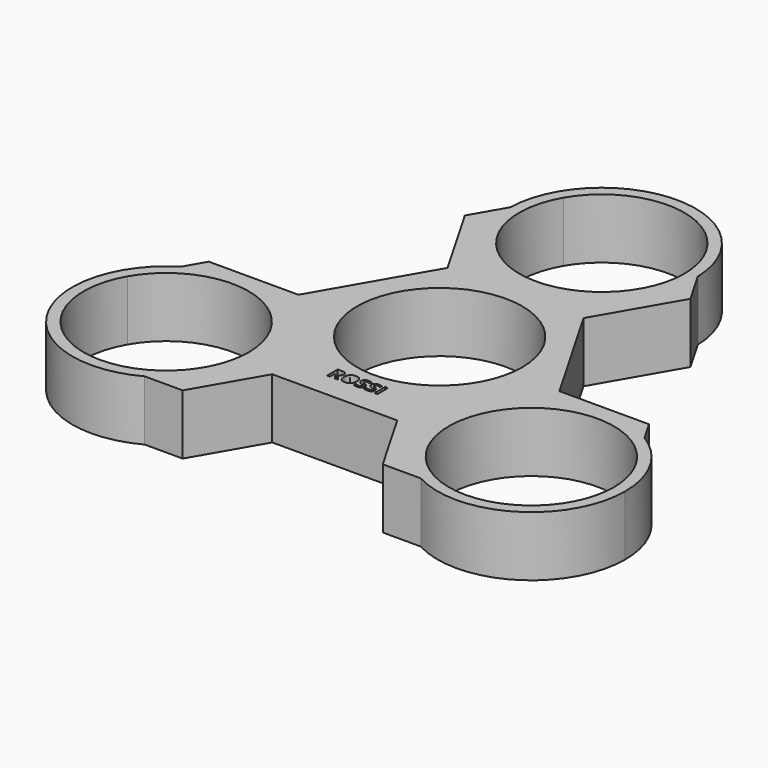
from build123d import *

# Parameters (mm, degrees)
F0_W     = 0.3740603024
F0_H     = 1.7637580204
F0_R     = 11
F1_DEPTH = 8


with BuildPart() as f1:
    # F0 (on Top) → F1 (new body)
    with BuildSketch(Plane.XY):
        with BuildLine():
            ThreePointArc((9.5262794416, 32.5), (10.6251840892, 29.8470094961), (11, 27))
            ThreePointArc((11, 27), (-2.8470094961, 16.3748159108), (-9.5262794416, 32.5))
            Line((-9.5262794416, 32.5), (-12.4948649634, 27.3582590497))
            ThreePointArc((-12.4948649634, 27.3582590497), (-0.1791479244, 14.5012838251), (12.5, 27))
            ThreePointArc((12.5, 27), (12.4987161749, 27.1791479244), (12.4948649634, 27.3582590497))
            Line((12.4948649634, 27.3582590497), (9.5262794416, 32.5))
        make_face()
        with BuildLine():
            ThreePointArc((-9.5262794416, 32.5), (0, 38), (9.5262794416, 32.5))
            Line((9.5262794416, 32.5), (12.4948649634, 27.3582590497))
            ThreePointArc((12.4948649634, 27.3582590497), (0, 39.5), (-12.4948649634, 27.3582590497))
            Line((-12.4948649634, 27.3582590497), (-9.5262794416, 32.5))
        make_face()
        with BuildLine():
            Line((15.0262794416, 22.9737205584), (12.4948649634, 27.3582590497))
            ThreePointArc((12.4948649634, 27.3582590497), (12.4987161749, 27.1791479244), (12.5, 27))
            ThreePointArc((12.5, 27), (-0.1791479244, 14.5012838251), (-12.4948649634, 27.3582590497))
            Line((-12.4948649634, 27.3582590497), (-15.0262794416, 22.9737205584))
            Line((-15.0262794416, 22.9737205584), (-14.056548526, 21.2940973429))
            Line((-14.056548526, 21.2940973429), (-9.056548526, 12.633843305))
            Line((-9.056548526, 12.633843305), (-17.3833487871, -1.7885978117))
            Line((-17.3833487871, -1.7885978117), (-25.1564458013, -1.7885978117))
            Line((-25.1564458013, -1.7885978117), (-27.3833487871, -1.7885978117))
            Line((-27.3833487871, -1.7885978117), (-29.3228106184, -1.7885978117))
            Line((-29.3228106184, -1.7885978117), (-30.884494181, -4.4935130875))
            ThreePointArc((-30.884494181, -4.4935130875), (-18.2325888272, -4.2214743535), (-11.8268002611, -15.1352540378))
            ThreePointArc((-11.8268002611, -15.1352540378), (-13.5921685012, -21.5397587789), (-18.3896292176, -26.1352540378))
            Line((-18.3896292176, -26.1352540378), (-13.3268002611, -26.1352540378))
            Line((-13.3268002611, -26.1352540378), (-8.3268002611, -17.475))
            Line((-8.3268002611, -17.475), (8.3268002611, -17.475))
            Line((8.3268002611, -17.475), (13.3268002611, -26.1352540378))
            Line((13.3268002611, -26.1352540378), (18.3896292176, -26.1352540378))
            ThreePointArc((18.3896292176, -26.1352540378), (13.5014827138, -8.8852540378), (30.884494181, -4.4935130875))
            Line((30.884494181, -4.4935130875), (29.3228106184, -1.7885978117))
            Line((29.3228106184, -1.7885978117), (27.3833487871, -1.7885978117))
            Line((27.3833487871, -1.7885978117), (17.3833487871, -1.7885978117))
            Line((17.3833487871, -1.7885978117), (9.056548526, 12.633843305))
            Line((9.056548526, 12.633843305), (14.056548526, 21.2940973429))
            Line((14.056548526, 21.2940973429), (15.0262794416, 22.9737205584))
        make_face()
        with BuildLine():
            Line((-3.1034472328, -13.4669476308), (-3.3022512119, -13.4669476308))
            Line((-3.3022512119, -13.4669476308), (-3.3022512119, -14.143653214))
            Line((-3.3022512119, -14.143653214), (-3.6763115143, -14.143653214))
            Line((-3.6763115143, -14.143653214), (-3.6763115143, -12.3798951936))
            Line((-3.6763115143, -12.3798951936), (-3.1625093858, -12.3798951936))
            add(Edge.make_bspline(
                [(-3.1625093858, -12.3798951936), (-2.8027320877, -12.3798951936), (-2.630370968, -12.5107583954)],
                knots=[0, 0, 0, 1, 1, 1], degree=2))
            add(Edge.make_bspline(
                [(-2.630370968, -12.5107583954), (-2.4580098482, -12.6416215971), (-2.4580098482, -12.9083663536)],
                knots=[0, 0, 0, 1, 1, 1], degree=2))
            add(Edge.make_bspline(
                [(-2.4580098482, -12.9083663536), (-2.4580098482, -13.0639352925), (-2.5435148606, -13.1851478157)],
                knots=[0, 0, 0, 1, 1, 1], degree=2))
            add(Edge.make_bspline(
                [(-2.5435148606, -13.1851478157), (-2.629019873, -13.3063603389), (-2.7861329205, -13.3750731705)],
                knots=[0, 0, 0, 1, 1, 1], degree=2))
            add(Edge.make_bspline(
                [(-2.7861329205, -13.3750731705), (-2.3877529081, -13.9699409992), (-2.2673124392, -14.143653214)],
                knots=[0, 0, 0, 1, 1, 1], degree=2))
            Line((-2.2673124392, -14.143653214), (-2.6822916188, -14.143653214))
            Line((-2.6822916188, -14.143653214), (-3.1034472328, -13.4669476308))
        make_face(mode=Mode.SUBTRACT)
        with BuildLine():
            add(Edge.make_bspline(
                [(-0.6598954121, -12.586226702), (-0.4444922658, -12.8203521648), (-0.4444922658, -13.2592650273)],
                knots=[0, 0, 0, 1, 1, 1], degree=2))
            add(Edge.make_bspline(
                [(-0.4444922658, -13.2592650273), (-0.4444922658, -13.6974058357), (-0.6616325342, -13.9326893798)],
                knots=[0, 0, 0, 1, 1, 1], degree=2))
            add(Edge.make_bspline(
                [(-0.6616325342, -13.9326893798), (-0.8787728026, -14.167972924), (-1.2841013037, -14.167972924)],
                knots=[0, 0, 0, 1, 1, 1], degree=2))
            add(Edge.make_bspline(
                [(-1.2841013037, -14.167972924), (-1.6894298048, -14.167972924), (-1.9065700732, -13.9326893798)],
                knots=[0, 0, 0, 1, 1, 1], degree=2))
            add(Edge.make_bspline(
                [(-1.9065700732, -13.9326893798), (-2.1237103416, -13.6974058357), (-2.1237103416, -13.2569488645)],
                knots=[0, 0, 0, 1, 1, 1], degree=2))
            add(Edge.make_bspline(
                [(-2.1237103416, -13.2569488645), (-2.1237103416, -12.8164918933), (-1.9059910325, -12.5842965663)],
                knots=[0, 0, 0, 1, 1, 1], degree=2))
            add(Edge.make_bspline(
                [(-1.9059910325, -12.5842965663), (-1.6882717233, -12.3521012392), (-1.2817851408, -12.3521012392)],
                knots=[0, 0, 0, 1, 1, 1], degree=2))
            add(Edge.make_bspline(
                [(-1.2817851408, -12.3521012392), (-0.8752985583, -12.3521012392), (-0.6598954121, -12.586226702)],
                knots=[0, 0, 0, 1, 1, 1], degree=2))
        make_face(mode=Mode.SUBTRACT)
        with BuildLine():
            add(Edge.make_bspline(
                [(0.8705091999, -13.3625272883), (0.9621906465, -13.4812306351), (0.9621906465, -13.6537847684)],
                knots=[0, 0, 0, 1, 1, 1], degree=2))
            add(Edge.make_bspline(
                [(0.9621906465, -13.6537847684), (0.9621906465, -13.8927355705), (0.7902155539, -14.0303542472)],
                knots=[0, 0, 0, 1, 1, 1], degree=2))
            add(Edge.make_bspline(
                [(0.7902155539, -14.0303542472), (0.6182404613, -14.167972924), (0.3121209362, -14.167972924)],
                knots=[0, 0, 0, 1, 1, 1], degree=2))
            add(Edge.make_bspline(
                [(0.3121209362, -14.167972924), (0.0295490669, -14.167972924), (-0.1873981879, -14.0614294323)],
                knots=[0, 0, 0, 1, 1, 1], degree=2))
            Line((-0.1873981879, -14.0614294323), (-0.1873981879, -13.7140050028))
            add(Edge.make_bspline(
                [(-0.1873981879, -13.7140050028), (-0.0090536475, -13.7939126216), (0.1146680521, -13.8263389017)],
                knots=[0, 0, 0, 1, 1, 1], degree=2))
            add(Edge.make_bspline(
                [(0.1146680521, -13.8263389017), (0.2383897518, -13.8587651818), (0.341072972, -13.8587651818)],
                knots=[0, 0, 0, 1, 1, 1], degree=2))
            add(Edge.make_bspline(
                [(0.341072972, -13.8587651818), (0.4638296038, -13.8587651818), (0.5296472318, -13.8118628838)],
                knots=[0, 0, 0, 1, 1, 1], degree=2))
            add(Edge.make_bspline(
                [(0.5296472318, -13.8118628838), (0.5954648598, -13.7649605858), (0.5954648598, -13.6719280442)],
                knots=[0, 0, 0, 1, 1, 1], degree=2))
            add(Edge.make_bspline(
                [(0.5954648598, -13.6719280442), (0.5954648598, -13.6202004069), (0.5665128241, -13.5796675568)],
                knots=[0, 0, 0, 1, 1, 1], degree=2))
            add(Edge.make_bspline(
                [(0.5665128241, -13.5796675568), (0.5375607883, -13.5391347067), (0.4813938388, -13.5018830873)],
                knots=[0, 0, 0, 1, 1, 1], degree=2))
            add(Edge.make_bspline(
                [(0.4813938388, -13.5018830873), (0.4252268894, -13.4646314679), (0.2526727561, -13.3824076862)],
                knots=[0, 0, 0, 1, 1, 1], degree=2))
            add(Edge.make_bspline(
                [(0.2526727561, -13.3824076862), (0.0913134099, -13.3063603389), (0.0104407233, -13.2364894259)],
                knots=[0, 0, 0, 1, 1, 1], degree=2))
            add(Edge.make_bspline(
                [(0.0104407233, -13.2364894259), (-0.0704319633, -13.1666185128), (-0.1186853563, -13.0735859711)],
                knots=[0, 0, 0, 1, 1, 1], degree=2))
            add(Edge.make_bspline(
                [(-0.1186853563, -13.0735859711), (-0.1669387493, -12.9805534295), (-0.1669387493, -12.8566387163)],
                knots=[0, 0, 0, 1, 1, 1], degree=2))
            add(Edge.make_bspline(
                [(-0.1669387493, -12.8566387163), (-0.1669387493, -12.6223202399), (-0.0082815932, -12.4885618346)],
                knots=[0, 0, 0, 1, 1, 1], degree=2))
            add(Edge.make_bspline(
                [(-0.0082815932, -12.4885618346), (0.150375563, -12.3548034292), (0.4302452423, -12.3548034292)],
                knots=[0, 0, 0, 1, 1, 1], degree=2))
            add(Edge.make_bspline(
                [(0.4302452423, -12.3548034292), (0.5676709055, -12.3548034292), (0.6925506865, -12.3872297093)],
                knots=[0, 0, 0, 1, 1, 1], degree=2))
            add(Edge.make_bspline(
                [(0.6925506865, -12.3872297093), (0.8174304676, -12.4196559894), (0.9536980494, -12.4787181424)],
                knots=[0, 0, 0, 1, 1, 1], degree=2))
            Line((0.9536980494, -12.4787181424), (0.8332575805, -12.7697826089))
            add(Edge.make_bspline(
                [(0.8332575805, -12.7697826089), (0.6919716458, -12.7118785373), (0.5997111584, -12.6889099223)],
                knots=[0, 0, 0, 1, 1, 1], degree=2))
            add(Edge.make_bspline(
                [(0.5997111584, -12.6889099223), (0.507450671, -12.6659413072), (0.4182784008, -12.6659413072)],
                knots=[0, 0, 0, 1, 1, 1], degree=2))
            add(Edge.make_bspline(
                [(0.4182784008, -12.6659413072), (0.3121209362, -12.6659413072), (0.2553749461, -12.7153527816)],
                knots=[0, 0, 0, 1, 1, 1], degree=2))
            add(Edge.make_bspline(
                [(0.2553749461, -12.7153527816), (0.1986289559, -12.764764256), (0.1986289559, -12.8442858477)],
                knots=[0, 0, 0, 1, 1, 1], degree=2))
            add(Edge.make_bspline(
                [(0.1986289559, -12.8442858477), (0.1986289559, -12.8936973221), (0.221597571, -12.9305629143)],
                knots=[0, 0, 0, 1, 1, 1], degree=2))
            add(Edge.make_bspline(
                [(0.221597571, -12.9305629143), (0.2445661861, -12.9674285066), (0.2945567012, -13.0017849224)],
                knots=[0, 0, 0, 1, 1, 1], degree=2))
            add(Edge.make_bspline(
                [(0.2945567012, -13.0017849224), (0.3445472163, -13.0361413382), (0.531384354, -13.1253136084)],
                knots=[0, 0, 0, 1, 1, 1], degree=2))
            add(Edge.make_bspline(
                [(0.531384354, -13.1253136084), (0.7788277532, -13.2438239416), (0.8705091999, -13.3625272883)],
                knots=[0, 0, 0, 1, 1, 1], degree=2))
        make_face(mode=Mode.SUBTRACT)
        with BuildLine():
            add(Edge.make_bspline(
                [(2.231254882, -13.3625272883), (2.3229363287, -13.4812306351), (2.3229363287, -13.6537847684)],
                knots=[0, 0, 0, 1, 1, 1], degree=2))
            add(Edge.make_bspline(
                [(2.3229363287, -13.6537847684), (2.3229363287, -13.8927355705), (2.1509612361, -14.0303542472)],
                knots=[0, 0, 0, 1, 1, 1], degree=2))
            add(Edge.make_bspline(
                [(2.1509612361, -14.0303542472), (1.9789861435, -14.167972924), (1.6728666184, -14.167972924)],
                knots=[0, 0, 0, 1, 1, 1], degree=2))
            add(Edge.make_bspline(
                [(1.6728666184, -14.167972924), (1.3902947491, -14.167972924), (1.1733474942, -14.0614294323)],
                knots=[0, 0, 0, 1, 1, 1], degree=2))
            Line((1.1733474942, -14.0614294323), (1.1733474942, -13.7140050028))
            add(Edge.make_bspline(
                [(1.1733474942, -13.7140050028), (1.3516920347, -13.7939126216), (1.4754137343, -13.8263389017)],
                knots=[0, 0, 0, 1, 1, 1], degree=2))
            add(Edge.make_bspline(
                [(1.4754137343, -13.8263389017), (1.5991354339, -13.8587651818), (1.7018186542, -13.8587651818)],
                knots=[0, 0, 0, 1, 1, 1], degree=2))
            add(Edge.make_bspline(
                [(1.7018186542, -13.8587651818), (1.824575286, -13.8587651818), (1.890392914, -13.8118628838)],
                knots=[0, 0, 0, 1, 1, 1], degree=2))
            add(Edge.make_bspline(
                [(1.890392914, -13.8118628838), (1.956210542, -13.7649605858), (1.956210542, -13.6719280442)],
                knots=[0, 0, 0, 1, 1, 1], degree=2))
            add(Edge.make_bspline(
                [(1.956210542, -13.6719280442), (1.956210542, -13.6202004069), (1.9272585062, -13.5796675568)],
                knots=[0, 0, 0, 1, 1, 1], degree=2))
            add(Edge.make_bspline(
                [(1.9272585062, -13.5796675568), (1.8983064704, -13.5391347067), (1.842139521, -13.5018830873)],
                knots=[0, 0, 0, 1, 1, 1], degree=2))
            add(Edge.make_bspline(
                [(1.842139521, -13.5018830873), (1.7859725716, -13.4646314679), (1.6134184383, -13.3824076862)],
                knots=[0, 0, 0, 1, 1, 1], degree=2))
            add(Edge.make_bspline(
                [(1.6134184383, -13.3824076862), (1.4520590921, -13.3063603389), (1.3711864055, -13.2364894259)],
                knots=[0, 0, 0, 1, 1, 1], degree=2))
            add(Edge.make_bspline(
                [(1.3711864055, -13.2364894259), (1.2903137188, -13.1666185128), (1.2420603258, -13.0735859711)],
                knots=[0, 0, 0, 1, 1, 1], degree=2))
            add(Edge.make_bspline(
                [(1.2420603258, -13.0735859711), (1.1938069329, -12.9805534295), (1.1938069329, -12.8566387163)],
                knots=[0, 0, 0, 1, 1, 1], degree=2))
            add(Edge.make_bspline(
                [(1.1938069329, -12.8566387163), (1.1938069329, -12.6223202399), (1.352464089, -12.4885618346)],
                knots=[0, 0, 0, 1, 1, 1], degree=2))
            add(Edge.make_bspline(
                [(1.352464089, -12.4885618346), (1.5111212451, -12.3548034292), (1.7909909244, -12.3548034292)],
                knots=[0, 0, 0, 1, 1, 1], degree=2))
            add(Edge.make_bspline(
                [(1.7909909244, -12.3548034292), (1.9284165877, -12.3548034292), (2.0532963687, -12.3872297093)],
                knots=[0, 0, 0, 1, 1, 1], degree=2))
            add(Edge.make_bspline(
                [(2.0532963687, -12.3872297093), (2.1781761498, -12.4196559894), (2.3144437315, -12.4787181424)],
                knots=[0, 0, 0, 1, 1, 1], degree=2))
            Line((2.3144437315, -12.4787181424), (2.1940032627, -12.7697826089))
            add(Edge.make_bspline(
                [(2.1940032627, -12.7697826089), (2.052717328, -12.7118785373), (1.9604568406, -12.6889099223)],
                knots=[0, 0, 0, 1, 1, 1], degree=2))
            add(Edge.make_bspline(
                [(1.9604568406, -12.6889099223), (1.8681963532, -12.6659413072), (1.779024083, -12.6659413072)],
                knots=[0, 0, 0, 1, 1, 1], degree=2))
            add(Edge.make_bspline(
                [(1.779024083, -12.6659413072), (1.6728666184, -12.6659413072), (1.6161206283, -12.7153527816)],
                knots=[0, 0, 0, 1, 1, 1], degree=2))
            add(Edge.make_bspline(
                [(1.6161206283, -12.7153527816), (1.5593746381, -12.764764256), (1.5593746381, -12.8442858477)],
                knots=[0, 0, 0, 1, 1, 1], degree=2))
            add(Edge.make_bspline(
                [(1.5593746381, -12.8442858477), (1.5593746381, -12.8936973221), (1.5823432532, -12.9305629143)],
                knots=[0, 0, 0, 1, 1, 1], degree=2))
            add(Edge.make_bspline(
                [(1.5823432532, -12.9305629143), (1.6053118682, -12.9674285066), (1.6553023834, -13.0017849224)],
                knots=[0, 0, 0, 1, 1, 1], degree=2))
            add(Edge.make_bspline(
                [(1.6553023834, -13.0017849224), (1.7052928985, -13.0361413382), (1.8921300361, -13.1253136084)],
                knots=[0, 0, 0, 1, 1, 1], degree=2))
            add(Edge.make_bspline(
                [(1.8921300361, -13.1253136084), (2.1395734354, -13.2438239416), (2.231254882, -13.3625272883)],
                knots=[0, 0, 0, 1, 1, 1], degree=2))
        make_face(mode=Mode.SUBTRACT)
        with Locations((2.8295969551, -13.2617742038)):
            Rectangle(F0_W, F0_H, mode=Mode.SUBTRACT)
        Circle(F0_R, mode=Mode.SUBTRACT)
        with BuildLine():
            ThreePointArc((36.8268002611, -15.1352540378), (35.2405799455, -9.041042604), (30.884494181, -4.4935130875))
            Line((30.884494181, -4.4935130875), (33.8530797028, -9.6352540378))
            ThreePointArc((33.8530797028, -9.6352540378), (34.9519843503, -12.2882445417), (35.3268002611, -15.1352540378))
            ThreePointArc((35.3268002611, -15.1352540378), (32.1049748542, -22.9134286309), (24.3268002611, -26.1352540378))
            Line((24.3268002611, -26.1352540378), (18.3896292176, -26.1352540378))
            ThreePointArc((18.3896292176, -26.1352540378), (30.7313050022, -25.8698857978), (36.8268002611, -15.1352540378))
        make_face()
        with BuildLine():
            Line((33.8530797028, -9.6352540378), (30.884494181, -4.4935130875))
            ThreePointArc((30.884494181, -4.4935130875), (13.5014827138, -8.8852540378), (18.3896292176, -26.1352540378))
            Line((18.3896292176, -26.1352540378), (24.3268002611, -26.1352540378))
            ThreePointArc((24.3268002611, -26.1352540378), (14.8005208195, -9.6352540378), (33.8530797028, -9.6352540378))
        make_face()
        with BuildLine():
            ThreePointArc((-11.8268002611, -15.1352540378), (-18.2325888272, -4.2214743535), (-30.884494181, -4.4935130875))
            Line((-30.884494181, -4.4935130875), (-33.8530797028, -9.6352540378))
            ThreePointArc((-33.8530797028, -9.6352540378), (-21.479790765, -4.5100699487), (-13.3268002611, -15.1352540378))
            ThreePointArc((-13.3268002611, -15.1352540378), (-16.5486256681, -22.9134286309), (-24.3268002611, -26.1352540378))
            Line((-24.3268002611, -26.1352540378), (-18.3896292176, -26.1352540378))
            ThreePointArc((-18.3896292176, -26.1352540378), (-13.5921685012, -21.5397587789), (-11.8268002611, -15.1352540378))
        make_face()
        with BuildLine():
            Line((-33.8530797028, -9.6352540378), (-30.884494181, -4.4935130875))
            ThreePointArc((-30.884494181, -4.4935130875), (-35.1521178084, -21.3852540378), (-18.3896292176, -26.1352540378))
            Line((-18.3896292176, -26.1352540378), (-24.3268002611, -26.1352540378))
            ThreePointArc((-24.3268002611, -26.1352540378), (-33.8530797028, -20.6352540378), (-33.8530797028, -9.6352540378))
        make_face()
    extrude(amount=F1_DEPTH)


solid = f1.part
